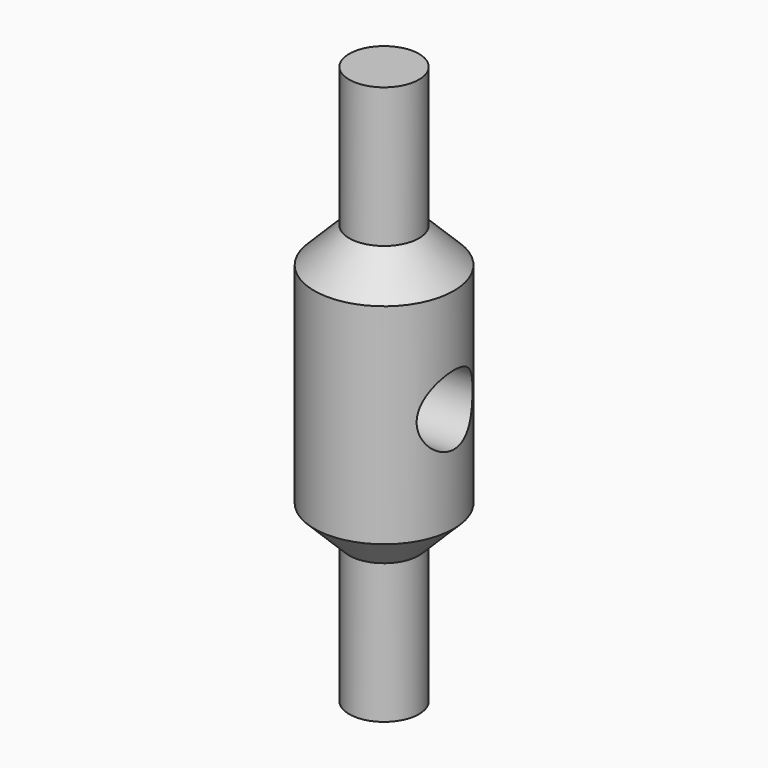
from build123d import *

# Parameters (mm, degrees)
F0_R     = 6.35
F1_DEPTH = 12.7
F2_R     = 3.175
F3_DEPTH = 25.4
F4_SIZE  = 3.17499
F5_R     = 3.175
F6_DEPTH = 12.7


# Not quite as in the source:
# - a fillet or chamfer is up to 0.001 mm smaller than in the source, because OpenCascade refuses the exact size


with BuildPart() as f1:
    # F0 (on Top) → F1 (new body, symmetric)
    with BuildSketch(Plane.XY):
        Circle(F0_R)
    extrude(amount=F1_DEPTH, both=True)

    # F2 (on Top) → F3 (join, symmetric)
    with BuildSketch(Plane.XY):
        Circle(F2_R)
    extrude(amount=F3_DEPTH, both=True)

    # F4 (size 3.175 in the source; OpenCascade refuses exactly that, so slightly less here)
    f4_edges = [f1.edges().sort_by_distance(p)[0] for p in [
        (-6.35, 0, -12.7),
        (-6.35, 0, 12.7),
    ]]
    chamfer(f4_edges, length=F4_SIZE)

    # F5 (on Right) → F6 (cut, symmetric)
    with BuildSketch(Plane.YZ):
        Circle(F5_R)
    extrude(amount=F6_DEPTH, both=True, mode=Mode.SUBTRACT)


solid = f1.part
